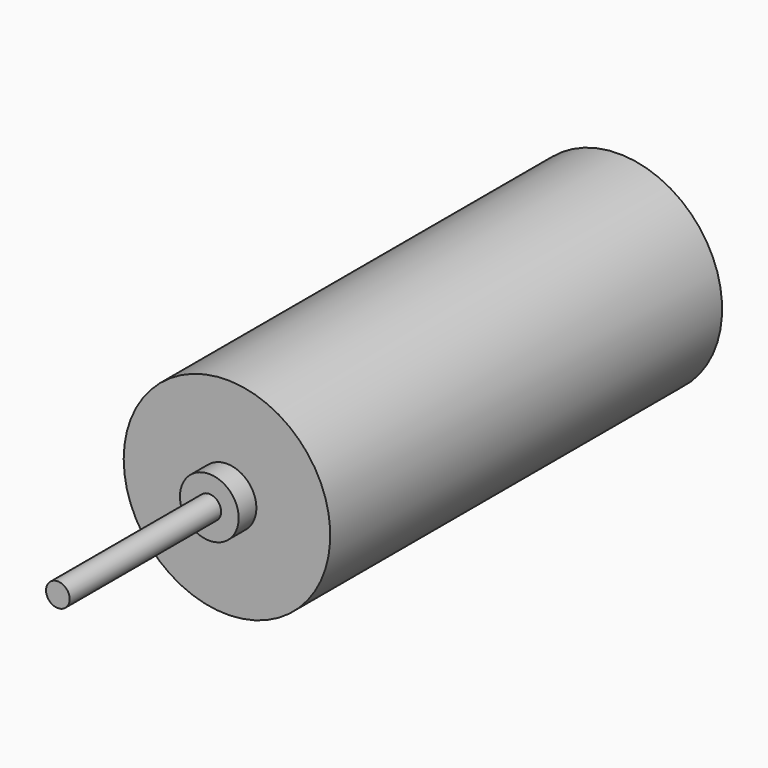
from build123d import *

# Parameters (mm, degrees)
F0_R     = 0.40005
F1_DEPTH = 6.4262
F2_R     = 0.99695
F2_R_2   = 0.40005
F3_DEPTH = 0.7493
F4_R     = 3.5052
F4_R_2   = 0.99695
F5_DEPTH = 16.6243
F6_R     = 0.92075
F7_DEPTH = 0.9525


with BuildPart() as f1:
    # F0 (on Front) → F1 (new body)
    with BuildSketch(Plane.XZ):
        Circle(F0_R)
    extrude(amount=-F1_DEPTH)

    # F2 (on face) → F3 (join)
    with BuildSketch(Plane(origin=(0, 6.4262, 0), x_dir=(-1, 0, 0), z_dir=(0, 1, 0))):
        Circle(F2_R)
        Circle(F2_R_2, mode=Mode.SUBTRACT)
        Circle(F2_R_2)
    extrude(amount=F3_DEPTH)

    # F4 (on face) → F5 (join)
    with BuildSketch(Plane(origin=(0, 7.1755, 0), x_dir=(-1, 0, 0), z_dir=(0, 1, 0))):
        Circle(F4_R)
        Circle(F4_R_2, mode=Mode.SUBTRACT)
        Circle(F4_R_2)
    extrude(amount=F5_DEPTH)

    # F6 (on face) → F7 (join)
    with BuildSketch(Plane(origin=(0, 23.7998, 0), x_dir=(-1, 0, 0), z_dir=(0, 1, 0))):
        Circle(F6_R)
    extrude(amount=F7_DEPTH)


solid = f1.part
